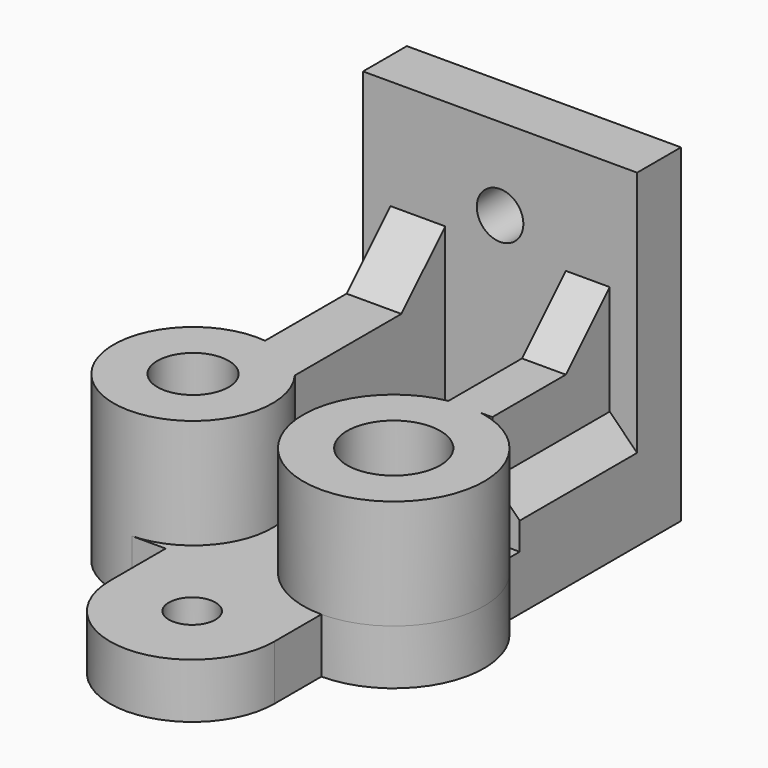
from build123d import *

# Parameters (mm, degrees)
F0_R          = 3.25
F0_R_2        = 2.125
F0_R_3        = 4.25
F1_DEPTH      = 5
F2_W          = 25
F2_H          = 5
F3_DEPTH      = 25
F4_R          = 7.25
F4_R_2        = 3.25
F4_R_3        = 8.25
F4_R_4        = 4.25
F5_DEPTH      = 10
F6_R          = 2.125
F7_DEPTH      = 5.001
F8_W          = 5
F8_H          = 17.15
F8_W_2        = 4
F8_H_2        = 13.3875096302
F9_DEPTH      = 10
F10_T1_DEPTH  = 5
F10_T3_DEPTH  = 4
F10_T8_DEPTH  = 30.7168298797
F10_T13_DEPTH = 29.7168298797
F10_T18_DEPTH = 27.1526880508
F10_S20_R     = 3.25
F10_T21_DEPTH = 16
F10_T25_DEPTH = 13.3875096302


# Not quite as in the source:
# - a fillet or chamfer that OpenCascade refuses, or shapes differently, is made with other operations: its cross-section is extruded or revolved along the edge and cut away or added


with BuildPart() as f1:
    # F0 (on Top) → F1 (new body)
    with BuildSketch(Plane.XY):
        with BuildLine():
            Line((12.5, 26.5), (0, 26.5))
            Line((0, 26.5), (-12.5, 26.5))
            Line((-12.5, 26.5), (-12.5, 7.0478720193))
            ThreePointArc((-12.5, 7.0478720193), (-17.9845104515, -0.9722703187), (-10.5656007648, -7.2462098368))
            Line((-10.5656007648, -7.2462098368), (-7.5, -7.2462098368))
            Line((-7.5, -7.2462098368), (-7.5, -13.6))
            ThreePointArc((-7.5, -13.6), (-5.3033008589, -18.9033008589), (0, -21.1))
            ThreePointArc((0, -21.1), (5.3033008589, -18.9033008589), (7.5, -13.6))
            Line((7.5, -13.6), (7.5, -8.25))
            ThreePointArc((7.5, -8.25), (15.3166703137, -2.6385915194), (12.5, 6.5622023742))
            Line((12.5, 6.5622023742), (12.5, 26.5))
        make_face()
        with Locations((-10.8, 0)):
            Circle(F0_R, mode=Mode.SUBTRACT)
        with Locations((0, -13.6)):
            Circle(F0_R_2, mode=Mode.SUBTRACT)
        with Locations((7.5, 0)):
            Circle(F0_R_3, mode=Mode.SUBTRACT)
        with Locations((0, 16.5)):
            Circle(F0_R_2, mode=Mode.SUBTRACT)
    extrude(amount=F1_DEPTH)

    # F2 (on face) → F3 (join)
    with BuildSketch(Plane.XY.offset(5)):
        with Locations((0, 24)):
            Rectangle(F2_W, F2_H)
    extrude(amount=F3_DEPTH)

    # F4 (on face) → F5 (join)
    with BuildSketch(Plane.XY.offset(5)):
        with Locations((-10.8, 0)):
            Circle(F4_R)
        with Locations((-10.8, 0)):
            Circle(F4_R_2, mode=Mode.SUBTRACT)
        with Locations((7.5, 0)):
            Circle(F4_R_3)
        with Locations((7.5, 0)):
            Circle(F4_R_4, mode=Mode.SUBTRACT)
    extrude(amount=F5_DEPTH)

    # F6 (on face) → F7 (cut, through all)
    with BuildSketch(Plane.XZ.offset(-21.5)):
        with Locations((0, 22.5)):
            Circle(F6_R)
    extrude(amount=-F7_DEPTH, mode=Mode.SUBTRACT)

    # F8 (on face) → F9 (join)
    with BuildSketch(Plane.XY.offset(5)):
        with Locations((-7.5, 12.925)):
            Rectangle(F8_W, F8_H)
        with Locations((8, 14.8062451849)):
            Rectangle(F8_W_2, F8_H_2)
    extrude(amount=F9_DEPTH)

    # F10: chamfer of 5 on 4 edges, made by hand

    # F10_s2 → F10_t1 (join)
    with BuildSketch(Plane.YZ.offset(-10)):
        Polygon((16.5, 15), (21.5, 20), (21.5, 15), align=None)
    extrude(amount=F10_T1_DEPTH)

    # F10_s4 → F10_t3 (join)
    with BuildSketch(Plane.YZ.offset(6)):
        Polygon((21.5, 20), (16.5, 15), (21.5, 15), align=None)
    extrude(amount=F10_T3_DEPTH)


with BuildPart() as f10_tool6:
    # F10_s7 → F10_t8 (new body)
    with BuildSketch(Plane.YZ.offset(7.8584149398)):
        Polygon((16.5, 15), (21.5, 20), (21.5, 15), align=None)
    extrude(amount=-F10_T8_DEPTH)

    split(bisect_by=Plane.YZ.offset(6), keep=Keep.TOP)


with BuildPart() as f1_1:
    add(f1.part)

    # F10_t5: union F10_tool6
    add(f10_tool6.part)


with BuildPart() as f10_tool11:
    # F10_s12 → F10_t13 (new body)
    with BuildSketch(Plane.YZ.offset(22.8584149398)):
        Polygon((21.5, 20), (16.5, 15), (21.5, 15), align=None)
    extrude(amount=-F10_T13_DEPTH)

    split(bisect_by=Plane.YZ.offset(-5), keep=Keep.BOTTOM)


with BuildPart() as f1_2:
    add(f1_1.part)

    # F10_t10: union F10_tool11
    add(f10_tool11.part)


with BuildPart() as f10_tool16:
    # F10_s17 → F10_t18 (new body)
    with BuildSketch(Plane.XZ.offset(-21.5)):
        Polygon((-10, 10), (-15, 5), (-10, 5), align=None)
    extrude(amount=F10_T18_DEPTH)

    split(bisect_by=Plane.YZ.offset(-12.5), keep=Keep.TOP)

    # F10_s20 → F10_t21 (cut, symmetric)
    with BuildSketch(Plane.XY.offset(7.5)):
        with Locations((-10.8, 0)):
            Circle(F10_S20_R)
    extrude(amount=F10_T21_DEPTH, both=True, mode=Mode.SUBTRACT)


with BuildPart() as f1_3:
    add(f1_2.part)

    # F10_t15: union F10_tool16
    add(f10_tool16.part)


with BuildPart() as f10_tool23:
    # F10_s24 → F10_t25 (new body)
    with BuildSketch(Plane.XZ.offset(-8.1124903698)):
        Polygon((10, 10), (15, 5), (10, 5), align=None)
    extrude(amount=-F10_T25_DEPTH)

    split(bisect_by=Plane.YZ.offset(12.5), keep=Keep.BOTTOM)


with BuildPart() as f1_4:
    add(f1_3.part)

    # F10_t22: union F10_tool23
    add(f10_tool23.part)


solid = f1_4.part
